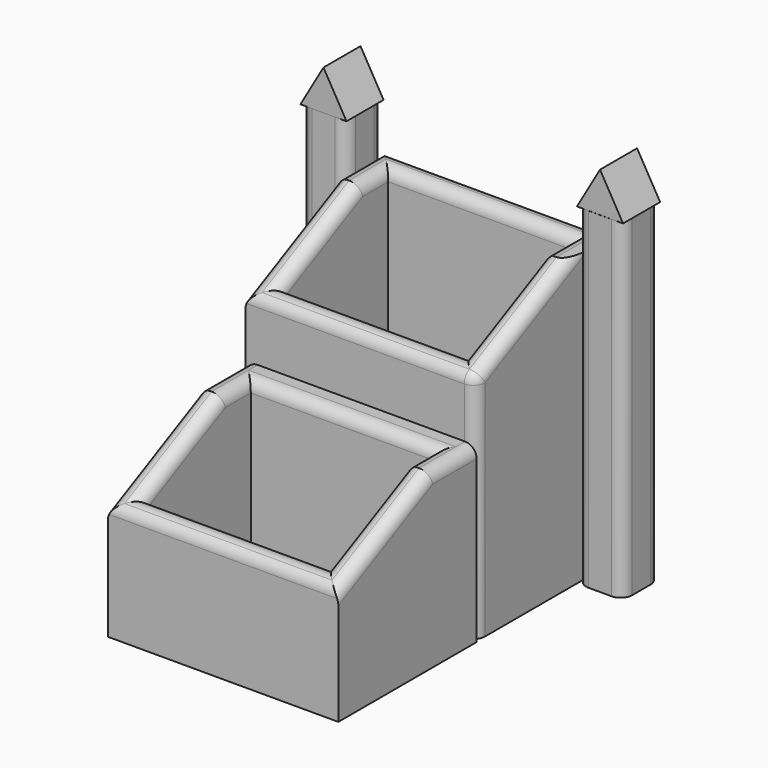
from build123d import *

# Parameters (mm, degrees)
F0_W           = 50.8
F0_H           = 38.1
F4_DEPTH       = 63.5
F1_W           = 50.8
F1_H           = 38.1
F5_DEPTH       = 38.1
F6_START       = 7.62
F2_W           = 40.64
F2_H           = 27.94
F6_DEPTH       = 55.88
F7_START       = 2.032
F3_W           = 40.64
F3_H           = 27.94
F7_DEPTH       = 59.182
F8_W           = 10.16
F8_H           = 10.16
F9_DEPTH       = 73.152
F11_START      = -51.562
F11_DEPTH      = 10.2108
F12_T1_DEPTH   = 182.3633067884
F12_2_T1_DEPTH = 182.3633067884
F13_R          = 2.53999
F13_2_R        = 2.53999
F13_3_R        = 2.53999
F13_4_R        = 2.53999


# Not quite as in the source:
# - a fillet or chamfer that OpenCascade refuses, or shapes differently, is made with other operations: its cross-section is extruded or revolved along the edge and cut away or added
# - a fillet or chamfer is up to 0.001 mm smaller than in the source, because OpenCascade refuses the exact size


with BuildPart() as f4:
    # F0 (on Top) → F4 (new body)
    with BuildSketch(Plane.XY):
        with Locations((-7.5105691367, 42.7431184798)):
            Rectangle(F0_W, F0_H)
    extrude(amount=F4_DEPTH)

    # F2 (on Top) → F6 (cut)
    with BuildSketch(Plane.XY.offset(F6_START)):
        with Locations((-7.5105691367, 42.7431184798)):
            Rectangle(F2_W, F2_H)
    extrude(amount=F6_DEPTH, mode=Mode.SUBTRACT)

    # F12: chamfer of 25.4 x 12.7 on 1 edges, made by hand

    # F12_s2 → F12_t1 (cut)
    with BuildSketch(Plane.YZ.offset(-98.6922225309)):
        Polygon((23.6931184798, 50.8), (49.0931184798, 63.5), (23.6931184798, 63.5), align=None)
    extrude(amount=F12_T1_DEPTH, mode=Mode.SUBTRACT)

    # F13 (radius 2.54 in the source; OpenCascade refuses exactly that, so slightly less here)
    f13_edges = [f4.edges().sort_by_distance(p)[0] for p in [
        (-7.510569, 28.773118, 53.34),
        (-27.830569, 38.933118, 58.42),
        (-27.830569, 52.903118, 63.5),
        (-7.510569, 56.713118, 63.5),
        (12.809431, 52.903118, 63.5),
        (12.809431, 38.933118, 58.42),
        (-32.910569, 36.393118, 57.15),
        (-7.510569, 61.793118, 63.5),
        (17.889431, 36.393118, 57.15),
        (-7.510569, 23.693118, 50.8),
        (-32.910569, 55.443118, 63.5),
        (17.889431, 23.693118, 25.4),
    ]]
    fillet(f13_edges, radius=F13_R)


with BuildPart() as f5:
    # F1 (on Top) → F5 (new body)
    with BuildSketch(Plane.XY):
        with Locations((-7.3355720048, 4.6431184798)):
            Rectangle(F1_W, F1_H)
    extrude(amount=F5_DEPTH)

    # F3 (on Top) → F7 (cut)
    with BuildSketch(Plane.XY.offset(F7_START)):
        with Locations((-7.3355720048, 4.6431184798)):
            Rectangle(F3_W, F3_H)
    extrude(amount=F7_DEPTH, mode=Mode.SUBTRACT)

    # F12#2: chamfer of 25.4 x 12.7 on 1 edges, made by hand

    # F12_2_s2 → F12_2_t1 (cut)
    with BuildSketch(Plane.YZ.offset(-98.517225399)):
        Polygon((-14.4068815202, 25.4), (10.9931184798, 38.1), (-14.4068815202, 38.1), align=None)
    extrude(amount=F12_2_T1_DEPTH, mode=Mode.SUBTRACT)

    # F13#2 (radius 2.54 in the source; OpenCascade refuses exactly that, so slightly less here)
    f13_2_edges = [f5.edges().sort_by_distance(p)[0] for p in [
        (-7.335572, 18.613118, 38.1),
        (-27.655572, 14.803118, 38.1),
        (-27.655572, 0.833118, 33.02),
        (12.984428, 0.833118, 33.02),
        (12.984428, 14.803118, 38.1),
        (-7.335572, -9.326882, 27.94),
        (18.064428, 17.343118, 38.1),
        (18.064428, -1.706882, 31.75),
        (-7.335572, -14.406882, 25.4),
        (-32.735572, -1.706882, 31.75),
        (-32.735572, 17.343118, 38.1),
    ]]
    fillet(f13_2_edges, radius=F13_2_R)


with BuildPart() as f9:
    # F8 (on Top) → F9 (new body)
    with BuildSketch(Plane.XY):
        with Locations((-37.9905691367, 56.6465079886)):
            Rectangle(F8_W, F8_H)
    extrude(amount=F9_DEPTH)

    # F13#3 (radius 2.54 in the source; OpenCascade refuses exactly that, so slightly less here)
    f13_3_edges = [f9.edges().sort_by_distance(p)[0] for p in [
        (-43.070569, 51.566508, 36.576),
        (-43.070569, 61.726508, 36.576),
        (-32.910569, 61.726508, 36.576),
        (-32.910569, 51.566508, 36.576),
    ]]
    fillet(f13_3_edges, radius=F13_3_R)


with BuildPart() as f9b:
    # F8 (on Top) → F9, piece 2 (new body)
    with BuildSketch(Plane.XY):
        with Locations((22.9694308633, 56.6185530889)):
            Rectangle(F8_W, F8_H)
    extrude(amount=F9_DEPTH)

    # F13#4 (radius 2.54 in the source; OpenCascade refuses exactly that, so slightly less here)
    f13_4_edges = [f9b.edges().sort_by_distance(p)[0] for p in [
        (28.049431, 61.698553, 36.576),
        (17.889431, 51.538553, 36.576),
        (28.049431, 51.538553, 36.576),
        (17.889431, 61.698553, 36.576),
    ]]
    fillet(f13_4_edges, radius=F13_4_R)


with BuildPart() as f11:
    # F10 (on Front) → F11 (new body)
    with BuildSketch(Plane.XZ.offset(F11_START)):
        Polygon((-37.9905691367, 81.9508181024), (-43.0705691367, 73.152), (-32.9105691367, 73.152), align=None)
    extrude(amount=-F11_DEPTH)


with BuildPart() as f11b:
    # F10 (on Front) → F11, piece 2 (new body)
    with BuildSketch(Plane.XZ.offset(F11_START)):
        Polygon((22.9694308633, 81.9508181024), (17.8894308633, 73.152), (28.0494308633, 73.152), align=None)
    extrude(amount=-F11_DEPTH)


solid = Compound([f4.part, f5.part, f9.part, f9b.part, f11.part, f11b.part])
